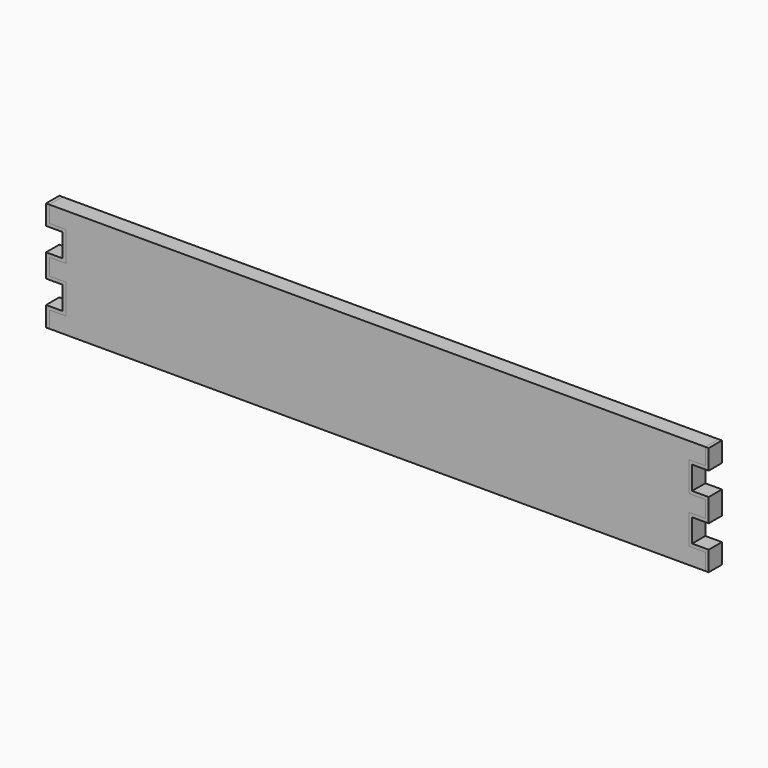
from build123d import *

# Parameters (mm, degrees)
F2_DEPTH = 5
F3_DEPTH = 5


with BuildPart() as f2:
    # F1 (on Front) → F2 (new body, symmetric)
    with BuildSketch(Plane.XZ):
        Polygon((0, 10), (0, 0), (198, 0), (396, 0), (396, 10), (386, 10), (386, 28), (396, 28), (396, 38), (386, 38), (386, 56), (396, 56), (396, 66), (198, 66), (0, 66), (0, 56), (10, 56), (10, 38), (0, 38), (0, 28), (10, 28), (10, 10), align=None)
    extrude(amount=F2_DEPTH, both=True)


with BuildPart() as f3:
    # F1 (on Front) → F3 (new body, symmetric)
    with BuildSketch(Plane.XZ):
        Polygon((-2, 0), (0, 0), (0, 10), (10, 10), (10, 28), (0, 28), (0, 38), (10, 38), (10, 56), (0, 56), (0, 66), (-2, 66), (-2, 54), (8, 54), (8, 40), (-2, 40), (-2, 26), (8, 26), (8, 12), (-2, 12), align=None)
    extrude(amount=F3_DEPTH, both=True)


with BuildPart() as f3b:
    # F1 (on Front) → F3, piece 2 (new body, symmetric)
    with BuildSketch(Plane.XZ):
        Polygon((396, 10), (396, 0), (398, 0), (398, 12), (388, 12), (388, 26), (398, 26), (398, 40), (388, 40), (388, 54), (398, 54), (398, 66), (396, 66), (396, 56), (386, 56), (386, 38), (396, 38), (396, 28), (386, 28), (386, 10), align=None)
    extrude(amount=F3_DEPTH, both=True)


solid = Compound([f2.part, f3.part, f3b.part])
